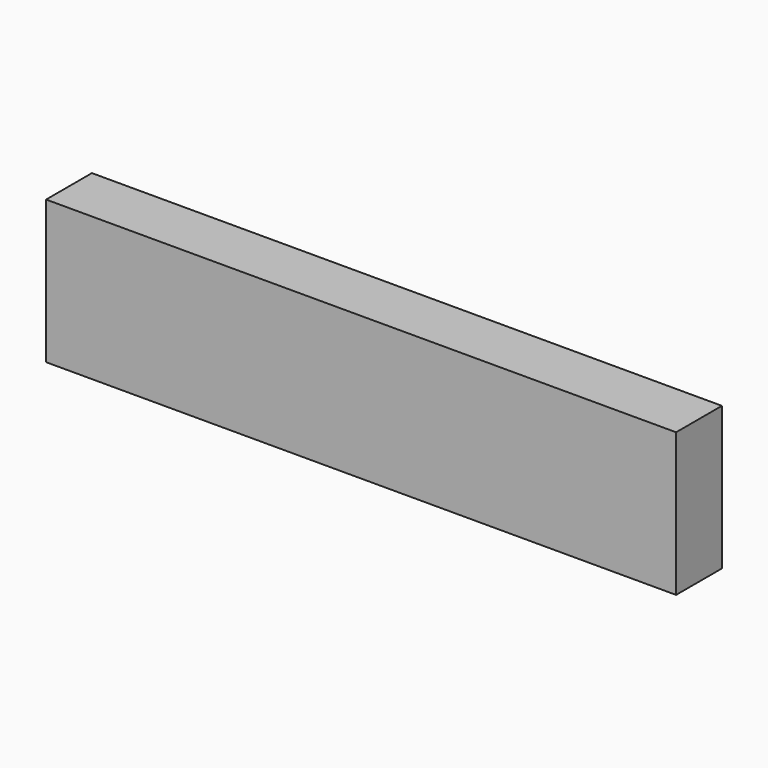
from build123d import *

# Parameters (mm, degrees)
F0_W     = 279.4
F0_H     = 63.5
F2_DEPTH = 25.4


# Not quite as in the source:
# - the program builds the solid bodies; features that only make, move or delete a surface that nothing else refers to are left out


with BuildPart() as f2:
    # F0 (on Front) → F2 (new body)
    with BuildSketch(Plane.XZ):
        Rectangle(F0_W, F0_H)
    extrude(amount=F2_DEPTH)


solid = f2.part
